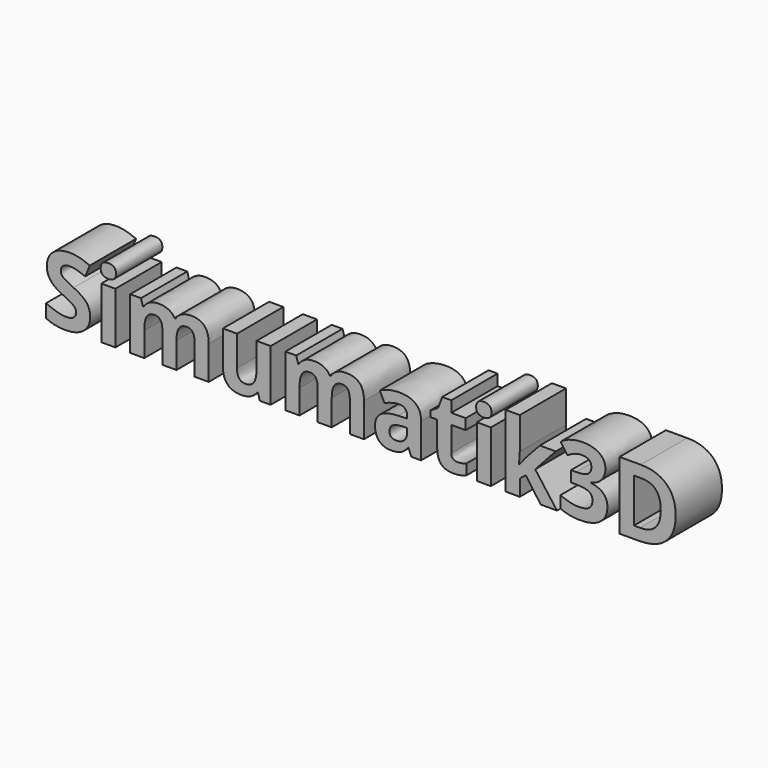
from build123d import *

# Parameters (mm, degrees)
F0_TEXT_SIZE = 32.7380715236
F1_DEPTH     = 20


# Not quite as in the source:
# - Text() gives the source's letters only with a copy of the font that has no kerning and outlines rounded to 1/6400 em; it was checked with that copy


with BuildPart() as f1:
    # F0 (on Front) → F1 (new body)
    with BuildSketch(Plane.XZ):
        with Locations((-102.9001707211, 0.0493224943)):
            Text('Simumatik3D', F0_TEXT_SIZE, font='Open Sans', font_style=FontStyle.BOLD, text_align=(TextAlign.LEFT, TextAlign.BOTTOM))
    extrude(amount=F1_DEPTH)


solid = f1.part
